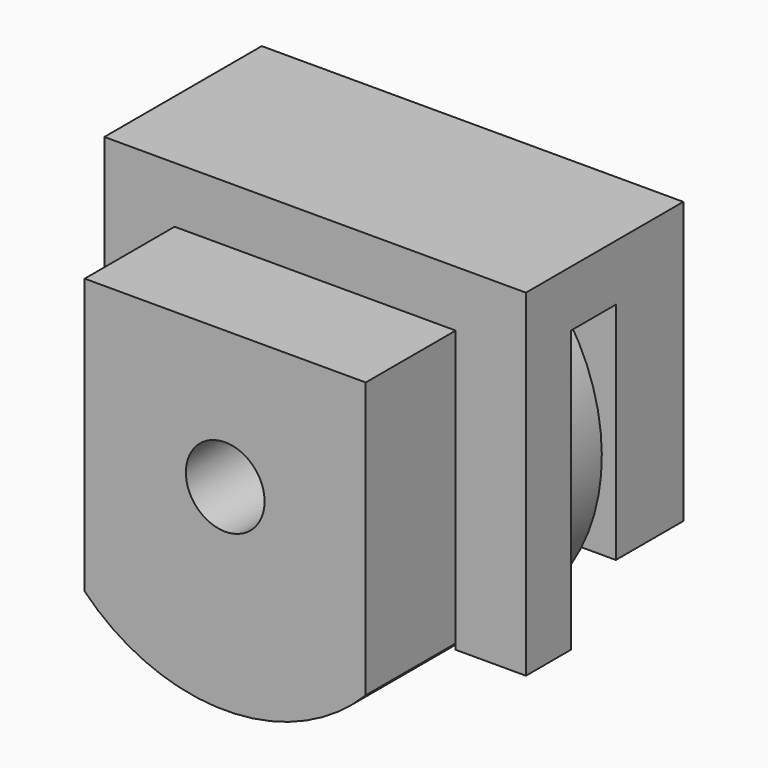
from build123d import *

# Parameters (mm, degrees)
F0_R      = 35
F0_R_2    = 7
F1_DEPTH  = 20
F2_W      = 10
F2_H      = 30
F3_DEPTH  = 35
F5_DEPTH  = 70
F6_R      = 17.5
F6_R_2    = 7
F7_DEPTH  = 9
F9_DEPTH  = 10
F11_DEPTH = 25
F12_W     = 75
F12_H     = 15
F13_DEPTH = 40
F14_W     = 24
F14_H     = 28.5051025722
F15_DEPTH = 25


# Not quite as in the source:
# - a feature names something its author has since deleted; it is built from what else it names


with BuildPart() as f1:
    # F0 (on Front) → F1 (new body, symmetric)
    with BuildSketch(Plane.XZ):
        Circle(F0_R)
        Circle(F0_R_2, mode=Mode.SUBTRACT)
    extrude(amount=F1_DEPTH, both=True)

    # F2 (on Top) → F3 (cut, symmetric)
    with BuildSketch(Plane.XY):
        with Locations((30, -5)):
            Rectangle(F2_W, F2_H)
        with Locations((-30, -5)):
            Rectangle(F2_W, F2_H)
    extrude(amount=F3_DEPTH, both=True, mode=Mode.SUBTRACT)

    # F4 (on face) → F5 (cut)
    with BuildSketch(Plane.YZ.offset(25)):
        Polygon((-20, 35), (-20, 24.4948974278), (10, 24.4948974278), (20, 24.4948974278), (20, 35), align=None)
    extrude(amount=-F5_DEPTH, mode=Mode.SUBTRACT)

    # F6 (on face) → F7 (cut)
    with BuildSketch(Plane(origin=(0, 20, 0), x_dir=(-1, 0, 0), z_dir=(0, 1, 0))):
        with Locations((-0.0028463546, -0.0477097929)):
            Circle(F6_R)
        Circle(F6_R_2, mode=Mode.SUBTRACT)
    extrude(amount=-F7_DEPTH, mode=Mode.SUBTRACT)


with BuildPart() as f9:
    # F8 (on face) → F9 (new body)
    with BuildSketch(Plane.XZ.offset(-10)):
        with BuildLine():
            ThreePointArc((25, -24.4948974278), (35, 0), (25, 24.4948974278))
            Line((25, 24.4948974278), (25, -24.4948974278))
        make_face()
        with BuildLine():
            Line((-37.5, 34.4948974278), (-37.5, -25.5051025722))
            Line((-37.5, -25.5051025722), (-25, -25.5051025722))
            Line((-25, -25.5051025722), (-25, 24.4948974278))
            Line((-25, 24.4948974278), (25, 24.4948974278))
            ThreePointArc((25, 24.4948974278), (35, 0), (25, -24.4948974278))
            Line((25, -24.4948974278), (25, -25.5051025722))
            Line((25, -25.5051025722), (37.5, -25.5051025722))
            Line((37.5, -25.5051025722), (37.5, 34.4948974278))
            Line((37.5, 34.4948974278), (-37.5, 34.4948974278))
        make_face()
    extrude(amount=F9_DEPTH)

    # F10 (on face) → F11 (join)
    with BuildSketch(Plane(origin=(0, 10, 0), x_dir=(-1, 0, 0), z_dir=(0, 1, 0))):
        Polygon((37.5, 34.4948974278), (-37.5, 34.4948974278), (-37.5, 24.4948974278), (-25, 24.4948974278), (25, 24.4948974278), (37.5, 24.4948974278), align=None)
    extrude(amount=F11_DEPTH)

    # F12 (on face) → F13 (join)
    with BuildSketch(Plane(origin=(0, 0, 24.4948974278), x_dir=(1, 0, 0), z_dir=(0, 0, -1))):
        with Locations((0, -27.5)):
            Rectangle(F12_W, F12_H)
    extrude(amount=F13_DEPTH)

    # F14 (on face) → F15 (cut)
    with BuildSketch(Plane(origin=(0, 35, 0), x_dir=(-1, 0, 0), z_dir=(0, 1, 0))):
        with Locations((0, -1.2525512861)):
            Rectangle(F14_W, F14_H)
    extrude(amount=-F15_DEPTH, mode=Mode.SUBTRACT)


solid = Compound([f1.part, f9.part])
